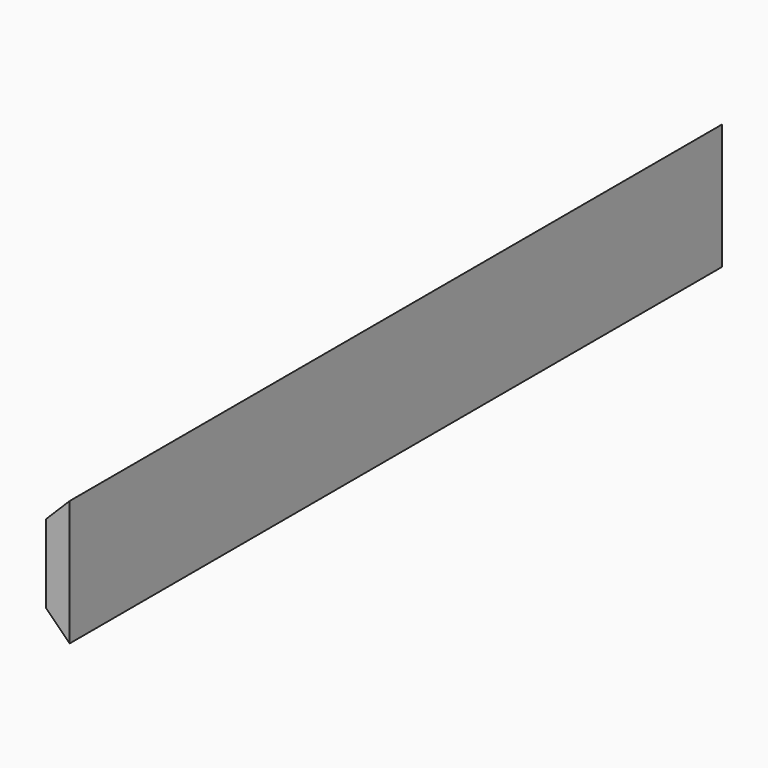
from build123d import *

# Parameters (mm, degrees)
F0_W     = 660.4
F0_H     = 101.6
F1_DEPTH = 19.05
F2_SIZE  = 19.04999


# Not quite as in the source:
# - a fillet or chamfer is up to 0.001 mm smaller than in the source, because OpenCascade refuses the exact size


with BuildPart() as f1:
    # F0 (on Right) → F1 (new body)
    with BuildSketch(Plane.YZ):
        with Locations((330.2, 50.8)):
            Rectangle(F0_W, F0_H)
    extrude(amount=F1_DEPTH)

    # F2 (size 19.05 in the source; OpenCascade refuses exactly that, so slightly less here)
    f2_edges = [f1.edges().sort_by_distance(p)[0] for p in [
        (0, 330.2, 101.6),
        (0, 330.2, 0),
    ]]
    chamfer(f2_edges, length=F2_SIZE)


solid = f1.part
